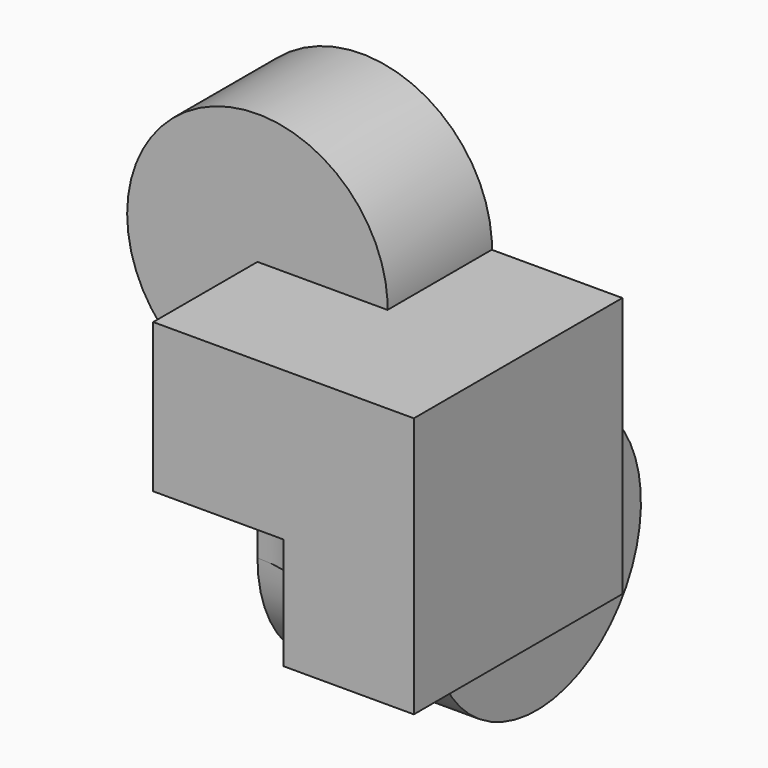
from build123d import *

# Parameters (mm, degrees)
F0_W     = 70
F0_H     = 70
F1_DEPTH = 70
F3_DEPTH = 29.972
F4_R     = 35
F5_DEPTH = 35
F6_R     = 35
F7_DEPTH = 46.99


with BuildPart() as f1:
    # F0 (on Top) → F1 (new body)
    with BuildSketch(Plane.XY):
        Rectangle(F0_W, F0_H)
    extrude(amount=F1_DEPTH)

    # F2 (on face) → F3 (cut)
    with BuildSketch(Plane(origin=(0, 0, 0), x_dir=(1, 0, 0), z_dir=(0, 0, -1))):
        with BuildLine():
            ThreePointArc((-35, 0), (-10.2512626585, 10.2512626585), (0, 35))
            Line((0, 35), (-35, 35))
            Line((-35, 35), (-35, 0))
        make_face()
    extrude(amount=-F3_DEPTH, mode=Mode.SUBTRACT)

    # F6 (on face) → F7 (join)
    with BuildSketch(Plane(origin=(-35, 0, 0), x_dir=(0, -1, 0), z_dir=(-1, 0, 0))):
        with Locations((-35, 0)):
            Circle(F6_R)
    extrude(amount=-F7_DEPTH)


with BuildPart() as f5:
    # F4 (on face) → F5 (new body)
    with BuildSketch(Plane(origin=(0, 35, 0), x_dir=(-1, 0, 0), z_dir=(0, 1, 0))):
        with Locations((35, 70)):
            Circle(F4_R)
    extrude(amount=-F5_DEPTH)


solid = Compound([f1.part, f5.part])
